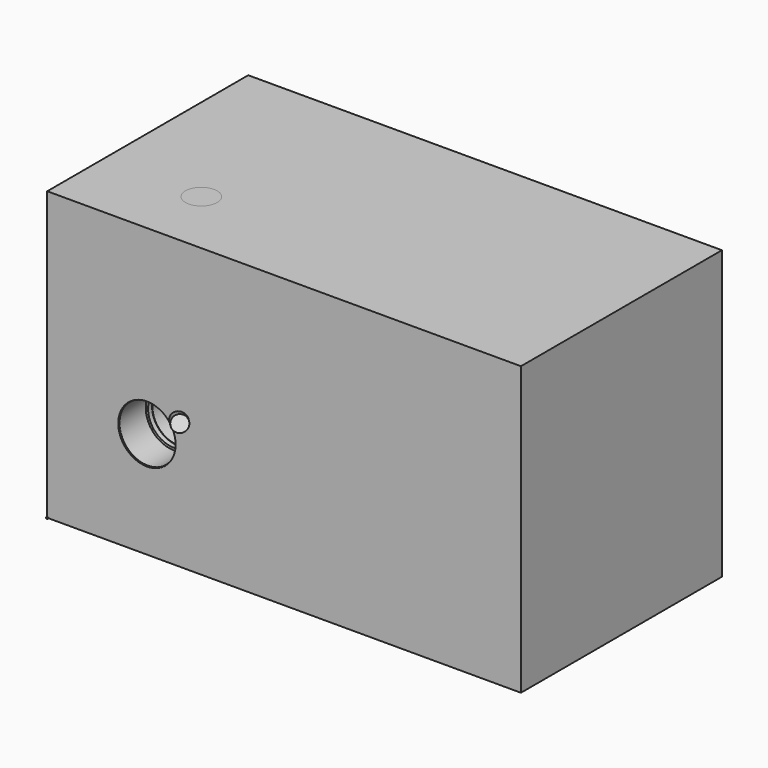
from build123d import *

# Parameters (mm, degrees)
F0_W      = 331.874368
F0_H      = 176.0200188
F1_DEPTH  = 201.4199934
F12_R     = 11.1125
F13_DEPTH = 138.111484
F14_R     = 20.09394
F15_DEPTH = 0.7874
F16_R     = 19.8501
F17_DEPTH = 21.4376
F18_R     = 19.8501
F19_DEPTH = 1.5748
F20_R     = 18.2753
F21_DEPTH = 3.2004
F22_R     = 18.2753
F23_DEPTH = 0.2794
F24_R     = 17.9959
F25_DEPTH = 17.9959
F26_R     = 17.9959
F27_DEPTH = 0.9144
F28_R     = 17.0815
F29_DEPTH = 18.1356
F37_R     = 5.2451
F38_DEPTH = 166.6868920692


with BuildPart() as f1:
    # F0 (on Top) → F1 (new body)
    with BuildSketch(Plane.XY):
        with Locations((165.937184, 88.0100094)):
            Rectangle(F0_W, F0_H)
    extrude(amount=F1_DEPTH)

    # F14 (on face) → F15 (cut)
    with BuildSketch(Plane.XZ):
        with Locations((69.85, 74.4210094)):
            Circle(F14_R)
    extrude(amount=-F15_DEPTH, mode=Mode.SUBTRACT)

    # F16 (on face) → F17 (cut)
    with BuildSketch(Plane.XZ.offset(-0.7874)):
        with Locations((69.85, 74.4210094)):
            Circle(F16_R)
    extrude(amount=-F17_DEPTH, mode=Mode.SUBTRACT)

    # F18 (on face) → F19 (cut)
    with BuildSketch(Plane.XZ.offset(-22.225)):
        with Locations((69.85, 74.4210094)):
            Circle(F18_R)
    extrude(amount=-F19_DEPTH, mode=Mode.SUBTRACT)

    # F20 (on face) → F21 (cut)
    with BuildSketch(Plane.XZ.offset(-23.7998)):
        with Locations((69.85, 74.4210094)):
            Circle(F20_R)
    extrude(amount=-F21_DEPTH, mode=Mode.SUBTRACT)

    # F22 (on face) → F23 (cut)
    with BuildSketch(Plane.XZ.offset(-27.0002)):
        with Locations((69.85, 74.4210094)):
            Circle(F22_R)
    extrude(amount=-F23_DEPTH, mode=Mode.SUBTRACT)

    # F24 (on face) → F25 (cut)
    with BuildSketch(Plane.XZ.offset(-27.2796)):
        with Locations((69.85, 74.4210094)):
            Circle(F24_R)
    extrude(amount=-F25_DEPTH, mode=Mode.SUBTRACT)

    # F26 (on face) → F27 (cut)
    with BuildSketch(Plane.XZ.offset(-45.2755)):
        with Locations((69.85, 74.4210094)):
            Circle(F26_R)
    extrude(amount=-F27_DEPTH, mode=Mode.SUBTRACT)

    # F28 (on face) → F29 (cut)
    with BuildSketch(Plane.XZ.offset(-46.1899)):
        with Locations((69.85, 74.4210094)):
            Circle(F28_R)
    extrude(amount=-F29_DEPTH, mode=Mode.SUBTRACT)


with BuildPart() as f3:
    # F2 (on Front) → F3 (revolve)
    with BuildSketch(Plane.XZ):
        with BuildLine():
            Line((0, 0.635), (0, -0.635))
            ThreePointArc((0, -0.635), (0.635, 0), (0, 0.635))
        make_face()
    revolve(axis=Axis((0, 0, 0), (0, 0, -1)))


with BuildPart() as f4_1:
    # F4: copy of F3
    add(f3.part.moved(Location((77.6531453284, 54.246543399, 157.1895892016))))


with BuildPart() as f5_1:
    # F5: copy of F3
    add(f3.part.moved(Location((64.2883685782, 39.0308466016, 125.9732336766))))


with BuildPart() as f6_1:
    # F6: copy of F3
    add(f3.part.moved(Location((77.6531453284, 54.246543399, 144.2983362186))))


with BuildPart() as f7_1:
    # F7: copy of F3
    add(f3.part.moved(Location((64.2883685782, 39.0308466016, 138.8644866596))))


with BuildPart() as f8_1:
    # F8: copy of F3
    add(f3.part.moved(Location((75.0607296598, 56.5236035134, 157.1895892016))))


with BuildPart() as f9_1:
    # F9: copy of F3
    add(f3.part.moved(Location((61.695952935, 41.3079067414, 125.9732336766))))


with BuildPart() as f10_1:
    # F10: copy of F3
    add(f3.part.moved(Location((75.0607296598, 56.5236035134, 144.2983362186))))


with BuildPart() as f11_1:
    # F11: copy of F3
    add(f3.part.moved(Location((61.695952935, 41.3079067414, 138.8644866596))))


with BuildPart() as f13:
    # F12 (on face) → F13 (new body)
    with BuildSketch(Plane.XY.offset(201.4199934)):
        with Locations((69.848984, 47.6240094)):
            Circle(F12_R)
    extrude(amount=-F13_DEPTH)


with BuildPart() as f38:
    # F37 (on line) → F38 (new body)
    with BuildSketch(Plane(origin=(-38.7516309373, 45.27287984, -22.5540213456), x_dir=(0.7938050593, 0.5443616512, -0.2711898237), z_dir=(0.6081722846, -0.7105174698, 0.3539652489))):
        with Locations((48.8175660776, 80.6456105024)):
            Circle(F37_R)
    extrude(amount=F38_DEPTH)


with BuildPart() as f39_1:
    # F39: copy of F3
    add(f3.part.moved(Location((70.7195639454, 33.7417338118, 69.1438927))))


with BuildPart() as f40_1:
    # F40: copy of F3
    add(f3.part.moved(Location((68.632947062, 31.9556793448, 69.1438927))))


with BuildPart() as f41_1:
    # F41: copy of F3
    add(f3.part.moved(Location((60.6933851916, 45.4551470626, 63.3085094))))


with BuildPart() as f42_1:
    # F42: copy of F3
    add(f3.part.moved(Location((58.6067683082, 43.6690925956, 63.3085094))))


with BuildPart() as f43_1:
    # F43: copy of F3
    add(f3.part.moved(Location((70.7195639454, 33.7417338118, 81.039212699))))


with BuildPart() as f44_1:
    # F44: copy of F3
    add(f3.part.moved(Location((68.632947062, 31.9556793448, 81.039212699))))


with BuildPart() as f45_1:
    # F45: copy of F3
    add(f3.part.moved(Location((56.2672708282, 50.6261007796, 72.6277658186))))


with BuildPart() as f46_1:
    # F46: copy of F3
    add(f3.part.moved(Location((54.1806539448, 48.840046338, 72.6277658186))))


with BuildPart() as f47_1:
    # F47: copy of F3
    add(f3.part.moved(Location((56.2672708282, 50.6261007796, 63.3085094))))


with BuildPart() as f48_1:
    # F48: copy of F3
    add(f3.part.moved(Location((54.1806539448, 48.840046338, 63.3085094))))


solid = Compound([f1.part, f3.part, f4_1.part, f5_1.part, f6_1.part, f7_1.part, f8_1.part, f9_1.part, f10_1.part, f11_1.part, f13.part, f38.part, f39_1.part, f40_1.part, f41_1.part, f42_1.part, f43_1.part, f44_1.part, f45_1.part, f46_1.part, f47_1.part, f48_1.part])
